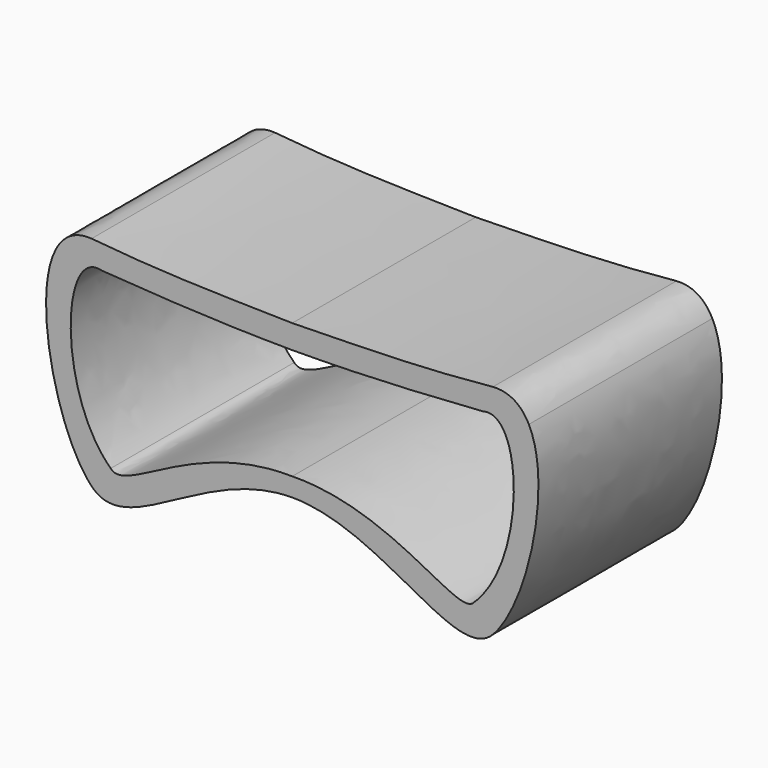
from build123d import *

# Parameters (mm, degrees)
F1_DEPTH = 400


with BuildPart() as f1:
    # F0 (on Front) → F1 (new body)
    with BuildSketch(Plane.XZ):
        with BuildLine():
            add(Edge.make_bspline(
                [(-349.9918261405, 164.7005370527), (-228.7541310859, 152.8680934101), (-148.4648335347, 151.7757154689), (0, 148.7712413073)],
                knots=[17.2755734709, 17.2755734709, 17.2755734709, 17.2755734709, 368.6136798781, 368.6136798781, 368.6136798781, 368.6136798781], degree=3))
            add(Edge.make_bspline(
                [(-349.9918261405, 164.7005370527), (-379.7747257767, 166.5833651071), (-400.0212253579, 152.0293008743), (-412.6107976831, 127.4847845064)],
                knots=[0, 0, 0, 0, 86.6035481416, 86.6035481416, 86.6035481416, 86.6035481416], degree=3))
            add(Edge.make_bspline(
                [(-412.6107976774, 127.4847845008), (-390.2805647898, 125.7630890537), (-367.6040024639, 124.021633923), (-344.5166107631, 122.3204635533)],
                knots=[55.3884070152, 55.3884070152, 55.3884070152, 55.3884070152, 129.1746995747, 129.1746995747, 129.1746995747, 129.1746995747], degree=3))
            add(Edge.make_bspline(
                [(-332.2621001683, 121.4244425258), (-336.5916827882, 122.5915718518), (-340.6786149646, 122.8620951072), (-344.5166107631, 122.3204635533)],
                knots=[0, 0, 0, 0, 17.888080119, 17.888080119, 17.888080119, 17.888080119], degree=3))
            add(Edge.make_bspline(
                [(-332.2621001683, 121.4244425258), (-231.2540764526, 114.0987320503), (-122.2665528935, 107.7345344123), (0, 107.2653010488)],
                knots=[142.1884395148, 142.1884395148, 142.1884395148, 142.1884395148, 462.9643141605, 462.9643141605, 462.9643141605, 462.9643141605], degree=3))
            add(Edge.make_bspline(
                [(332.2621001683, 121.4244425258), (231.2540764526, 114.0987320503), (122.2665528935, 107.7345344123), (0, 107.2653010488)],
                knots=[142.1884395148, 142.1884395148, 142.1884395148, 142.1884395148, 462.9643141605, 462.9643141605, 462.9643141605, 462.9643141605], degree=3))
            add(Edge.make_bspline(
                [(332.2621001683, 121.4244425258), (336.5916827882, 122.5915718518), (340.6786149646, 122.8620951072), (344.5166107631, 122.3204635533)],
                knots=[0, 0, 0, 0, 17.888080119, 17.888080119, 17.888080119, 17.888080119], degree=3))
            add(Edge.make_bspline(
                [(412.6107976774, 127.4847845008), (390.2805647898, 125.7630890537), (367.6040024639, 124.021633923), (344.5166107631, 122.3204635533)],
                knots=[55.3884070152, 55.3884070152, 55.3884070152, 55.3884070152, 129.1746995747, 129.1746995747, 129.1746995747, 129.1746995747], degree=3))
            add(Edge.make_bspline(
                [(349.9918261405, 164.7005370527), (379.7747257767, 166.5833651071), (400.0212253579, 152.0293008743), (412.6107976831, 127.4847845064)],
                knots=[0, 0, 0, 0, 86.6035481416, 86.6035481416, 86.6035481416, 86.6035481416], degree=3))
            add(Edge.make_bspline(
                [(349.9918261405, 164.7005370527), (228.7541310859, 152.8680934101), (148.4648335347, 151.7757154689), (0, 148.7712413073)],
                knots=[17.2755734709, 17.2755734709, 17.2755734709, 17.2755734709, 368.6136798781, 368.6136798781, 368.6136798781, 368.6136798781], degree=3))
        make_face()
        with BuildLine():
            add(Edge.make_bspline(
                [(-412.6107976774, 127.4847845008), (-390.2805647898, 125.7630890537), (-367.6040024639, 124.021633923), (-344.5166107631, 122.3204635533)],
                knots=[55.3884070152, 55.3884070152, 55.3884070152, 55.3884070152, 129.1746995747, 129.1746995747, 129.1746995747, 129.1746995747], degree=3))
            add(Edge.make_bspline(
                [(-412.6107976831, 127.4847845064), (-455.2641858876, 44.3281245427), (-410.0275390456, -153.5039344324), (-349.9918261405, -215.3152623841)],
                knots=[86.6035481416, 86.6035481416, 86.6035481416, 86.6035481416, 380.0157994368, 380.0157994368, 380.0157994368, 380.0157994368], degree=3))
            add(Edge.make_bspline(
                [(-349.9918261405, -215.3152623841), (-287.5397462749, -281.8407177446), (-155.7662200923, -118.8372276745), (0, -119.0087459604)],
                knots=[0, 0, 0, 0, 363.0003078109, 363.0003078109, 363.0003078109, 363.0003078109], degree=3))
            add(Edge.make_bspline(
                [(349.9918261405, -215.3152623841), (287.5397462749, -281.8407177446), (155.7662200923, -118.8372276745), (0, -119.0087459604)],
                knots=[0, 0, 0, 0, 363.0003078109, 363.0003078109, 363.0003078109, 363.0003078109], degree=3))
            add(Edge.make_bspline(
                [(412.6107976831, 127.4847845064), (455.2641858876, 44.3281245427), (410.0275390456, -153.5039344324), (349.9918261405, -215.3152623841)],
                knots=[86.6035481416, 86.6035481416, 86.6035481416, 86.6035481416, 380.0157994368, 380.0157994368, 380.0157994368, 380.0157994368], degree=3))
            add(Edge.make_bspline(
                [(412.6107976774, 127.4847845008), (390.2805647898, 125.7630890537), (367.6040024639, 124.021633923), (344.5166107631, 122.3204635533)],
                knots=[55.3884070152, 55.3884070152, 55.3884070152, 55.3884070152, 129.1746995747, 129.1746995747, 129.1746995747, 129.1746995747], degree=3))
            add(Edge.make_bspline(
                [(344.5166107631, 122.3204635533), (404.847274862, 113.8063866609), (403.6665423185, -95.3885912359), (316.5586292744, -177.2394478321)],
                knots=[17.888080119, 17.888080119, 17.888080119, 17.888080119, 299.0764424053, 299.0764424053, 299.0764424053, 299.0764424053], degree=3))
            add(Edge.make_bspline(
                [(316.5586292744, -177.2394478321), (289.4581258297, -209.2567682266), (174.6161052003, -83.5422830285), (0, -86.466948735)],
                knots=[0, 0, 0, 0, 329.3159764731, 329.3159764731, 329.3159764731, 329.3159764731], degree=3))
            add(Edge.make_bspline(
                [(-316.5586292744, -177.2394478321), (-289.4581258297, -209.2567682266), (-174.6161052003, -83.5422830285), (0, -86.466948735)],
                knots=[0, 0, 0, 0, 329.3159764731, 329.3159764731, 329.3159764731, 329.3159764731], degree=3))
            add(Edge.make_bspline(
                [(-344.5166107631, 122.3204635533), (-404.847274862, 113.8063866609), (-403.6665423185, -95.3885912359), (-316.5586292744, -177.2394478321)],
                knots=[17.888080119, 17.888080119, 17.888080119, 17.888080119, 299.0764424053, 299.0764424053, 299.0764424053, 299.0764424053], degree=3))
        make_face()
    extrude(amount=F1_DEPTH)


solid = f1.part
